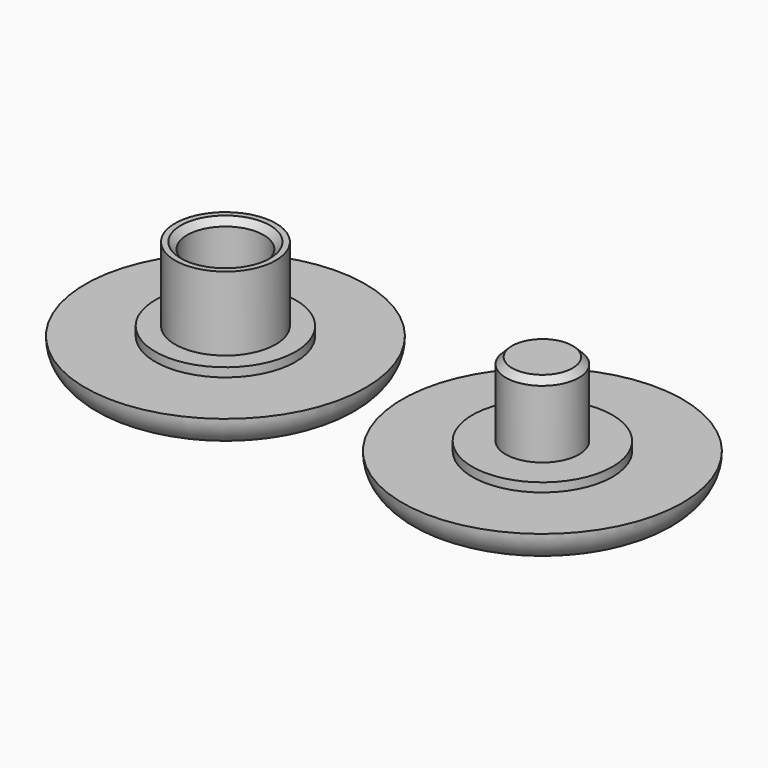
from build123d import *

# Parameters (mm, degrees)
F0_R     = 11
F0_R_2   = 5.5
F1_DEPTH = 2.5
F0_R_3   = 3.95
F2_DEPTH = 3.2
F0_R_4   = 3
F3_DEPTH = 9
F4_R     = 2.49999
F5_DEPTH = 2.5
F6_DEPTH = 2.5
F7_DEPTH = 3.2
F0_R_5   = 2.875
F8_DEPTH = 3.2
F9_DEPTH = 9
F10_R    = 2.49999
F11_SIZE = 0.5
F12_SIZE = 0.5


# Not quite as in the source:
# - a fillet or chamfer is up to 0.001 mm smaller than in the source, because OpenCascade refuses the exact size


with BuildPart() as f1:
    # F0 (on Top) → F1 (new body)
    with BuildSketch(Plane.XY):
        Circle(F0_R)
        Circle(F0_R_2, mode=Mode.SUBTRACT)
    extrude(amount=F1_DEPTH)

    # F0 (on Top) → F2 (join)
    with BuildSketch(Plane.XY):
        Circle(F0_R_2)
        Circle(F0_R_3, mode=Mode.SUBTRACT)
    extrude(amount=F2_DEPTH)

    # F0 (on Top) → F3 (join)
    with BuildSketch(Plane.XY):
        Circle(F0_R_3)
        Circle(F0_R_4, mode=Mode.SUBTRACT)
    extrude(amount=F3_DEPTH)

    # F4 (radius 2.5 in the source; OpenCascade refuses exactly that, so slightly less here)
    f4_edges = [f1.edges().sort_by_distance(p)[0] for p in [
        (-11, 0, 0),
    ]]
    fillet(f4_edges, radius=F4_R)

    # F0 (on Top) → F5 (join)
    with BuildSketch(Plane.XY):
        Circle(F0_R_4)
    extrude(amount=F5_DEPTH)

    # F12
    f12_edges = [f1.edges().sort_by_distance(p)[0] for p in [
        (-3, 0, 9),
    ]]
    chamfer(f12_edges, length=F12_SIZE)


with BuildPart() as f6:
    # F0 (on Top) → F6 (new body)
    with BuildSketch(Plane.XY):
        with Locations((24.7028488666, 0.2105356252)):
            Circle(F0_R)
        with Locations((24.7028488666, 0.2105356252)):
            Circle(F0_R_2, mode=Mode.SUBTRACT)
    extrude(amount=F6_DEPTH)

    # F0 (on Top) → F7 (join)
    with BuildSketch(Plane.XY):
        with Locations((24.7028488666, 0.2105356252)):
            Circle(F0_R_2)
        with Locations((24.7028488666, 0.2105356252)):
            Circle(F0_R_3, mode=Mode.SUBTRACT)
    extrude(amount=F7_DEPTH)

    # F0 (on Top) → F8 (join)
    with BuildSketch(Plane.XY):
        with Locations((24.7028488666, 0.2105356252)):
            Circle(F0_R_3)
        with Locations((24.7028488666, 0.2105356252)):
            Circle(F0_R_5, mode=Mode.SUBTRACT)
    extrude(amount=F8_DEPTH)

    # F0 (on Top) → F9 (join)
    with BuildSketch(Plane.XY):
        with Locations((24.7028488666, 0.2105356252)):
            Circle(F0_R_5)
    extrude(amount=F9_DEPTH)

    # F10 (radius 2.5 in the source; OpenCascade refuses exactly that, so slightly less here)
    f10_edges = [f6.edges().sort_by_distance(p)[0] for p in [
        (13.702849, 0.210536, 0),
    ]]
    fillet(f10_edges, radius=F10_R)

    # F11
    f11_edges = [f6.edges().sort_by_distance(p)[0] for p in [
        (21.827849, 0.210536, 9),
    ]]
    chamfer(f11_edges, length=F11_SIZE)


solid = Compound([f1.part, f6.part])
